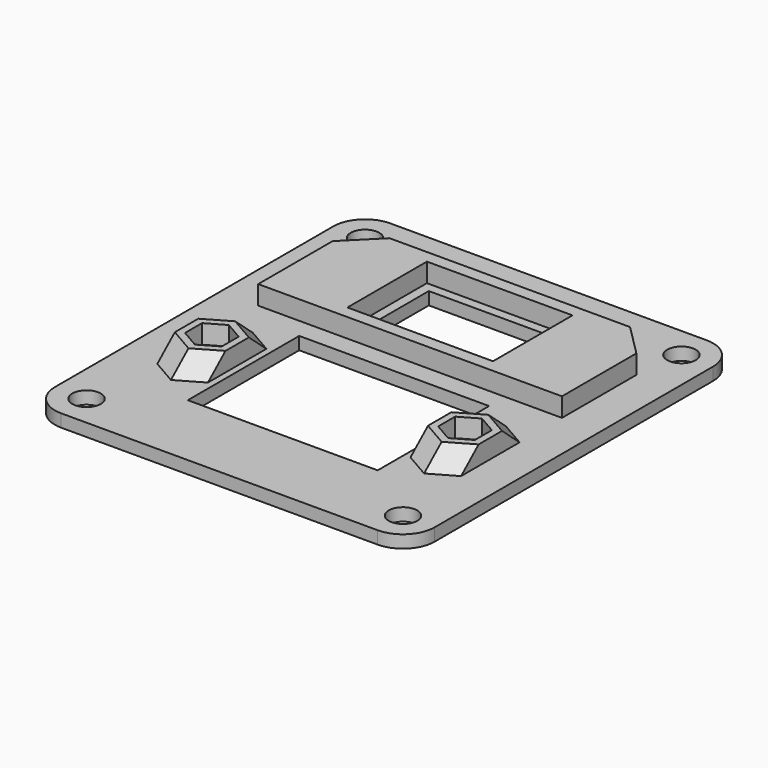
from build123d import *

# Parameters (mm, degrees)
F0_W      = 60
F0_H      = 65
F1_DEPTH  = 2
F2_W      = 20
F2_H      = 12.7
F3_DEPTH  = 25
F4_R      = 1.75
F4_W      = 30
F4_H      = 22
F5_DEPTH  = 25
F7_DEPTH  = 3
F8_SIZE   = 2.99999
F10_D     = 4.5
F11_R     = 5
F12_W     = 48
F12_H     = 19.7
F12_W_2   = 23
F12_H_2   = 15.7
F13_DEPTH = 3
F14_SIZE  = 5


# Not quite as in the source:
# - a fillet or chamfer is up to 0.001 mm smaller than in the source, because OpenCascade refuses the exact size
# - a pattern or mirror of a feature is missing from the dataset's text; its kind, count and spacing are read off the source's solid


with BuildPart() as f1:
    # F0 (on Top) → F1 (new body)
    with BuildSketch(Plane.XY):
        Rectangle(F0_W, F0_H)
    extrude(amount=F1_DEPTH)

    # F2 (on face) → F3 (cut)
    with BuildSketch(Plane.XY.offset(2)):
        with Locations((0, 15)):
            Rectangle(F2_W, F2_H)
    extrude(amount=-F3_DEPTH, mode=Mode.SUBTRACT)

    # F4 (on face) → F5 (cut)
    with BuildSketch(Plane.XY.offset(2)):
        with Locations((-20, -9)):
            Circle(F4_R)
        with Locations((0, -9)):
            Rectangle(F4_W, F4_H)
        with Locations((20, -9)):
            Circle(F4_R)
    extrude(amount=-F5_DEPTH, mode=Mode.SUBTRACT)

    # F6 (on face) → F7 (join)
    with BuildSketch(Plane.XY.offset(2)):
        Polygon((-24, -6.6905989232), (-24, -11.3094010768), (-20, -13.6188021535), (-16, -11.3094010768), (-16, -6.6905989232), (-20, -4.3811978465), align=None)
        Polygon((-20, -12.3486315613), (-22.9, -10.6743157806), (-22.9, -7.3256842194), (-20, -5.6513684387), (-17.1, -7.3256842194), (-17.1, -10.6743157806), align=None, mode=Mode.SUBTRACT)
    f7 = extrude(amount=F7_DEPTH)

    # F7_copies: F7 across plane
    add(f7.mirror(Plane(origin=(0, 0, 0), x_dir=(0, 0, 1), z_dir=(1, 0, 0))))

    # F8 (size 3 in the source; OpenCascade refuses exactly that, so slightly less here)
    f8_edges = [f1.edges().sort_by_distance(p)[0] for p in [
        (-22, -12.464102, 2),
        (-18, -12.464102, 2),
        (-22, -5.535898, 2),
        (-18, -5.535898, 2),
        (18, -5.535898, 2),
        (18, -12.464102, 2),
        (22, -12.464102, 2),
        (22, -5.535898, 2),
    ]]
    chamfer(f8_edges, length=F8_SIZE)

    # F10 (through all)
    with Locations(Plane.XY.offset(2)):
        with Locations((-25, 27.5), (25, 27.5), (25, -27.5), (-25, -27.5)):
            Hole(F10_D / 2)

    # F11
    f11_edges = [f1.edges().sort_by_distance(p)[0] for p in [
        (30, 32.5, 1),
        (-30, 32.5, 1),
        (30, -32.5, 1),
        (-30, -32.5, 1),
    ]]
    fillet(f11_edges, radius=F11_R)

    # F12 (on face) → F13 (join)
    with BuildSketch(Plane.XY.offset(2)):
        with Locations((0, 15)):
            Rectangle(F12_W, F12_H)
        with Locations((0, 15)):
            Rectangle(F12_W_2, F12_H_2, mode=Mode.SUBTRACT)
    extrude(amount=F13_DEPTH)

    # F14
    f14_edges = [f1.edges().sort_by_distance(p)[0] for p in [
        (24, 24.85, 3.5),
        (-24, 24.85, 3.5),
    ]]
    chamfer(f14_edges, length=F14_SIZE)


solid = f1.part
